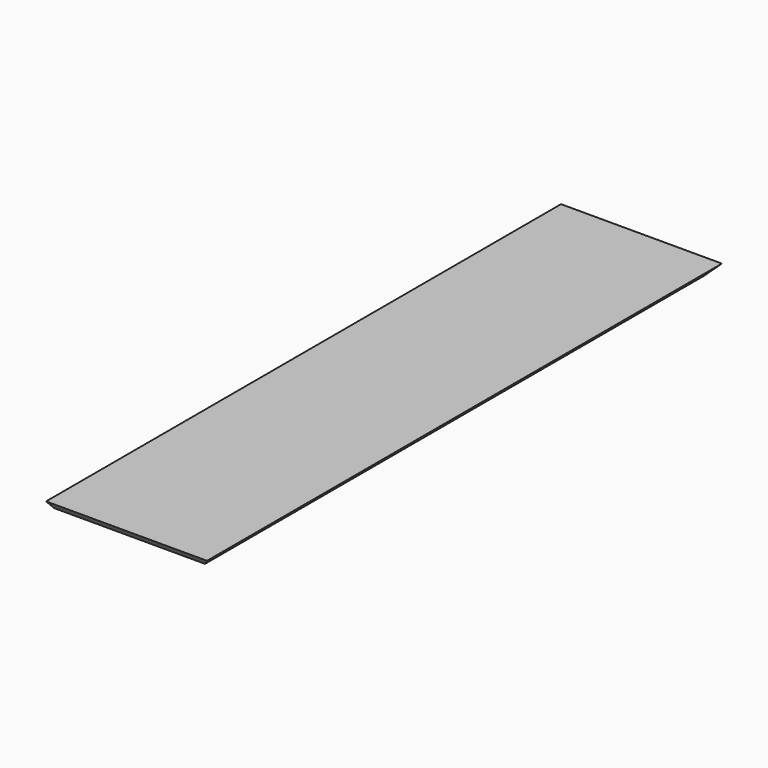
from build123d import *

# Parameters (mm, degrees)
F0_W     = 400
F0_H     = 1600
F1_DEPTH = 12.5
F2_SIZE  = 24.99999


# Not quite as in the source:
# - a fillet or chamfer is up to 0.001 mm smaller than in the source, because OpenCascade refuses the exact size


with BuildPart() as f1:
    # F0 (on Top) → F1 (new body, symmetric)
    with BuildSketch(Plane.XY):
        Rectangle(F0_W, F0_H)
    extrude(amount=F1_DEPTH, both=True)

    # F2 (size 25 in the source; OpenCascade refuses exactly that, so slightly less here)
    f2_edges = [f1.edges().sort_by_distance(p)[0] for p in [
        (0, -800, -12.5),
        (0, 800, -12.5),
        (200, 0, -12.5),
    ]]
    chamfer(f2_edges, length=F2_SIZE)


solid = f1.part
